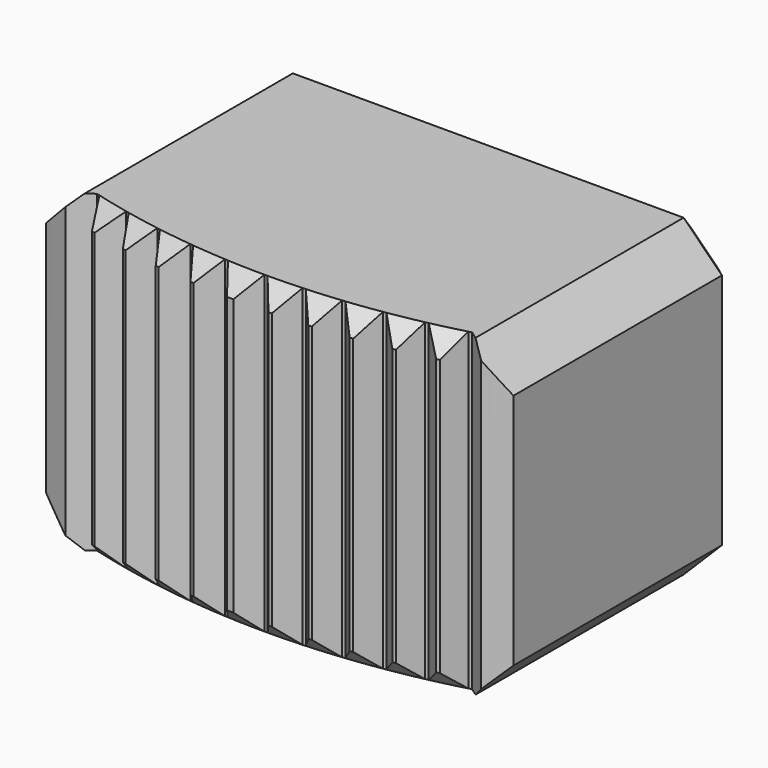
from build123d import *

# Parameters (mm, degrees)
F1_DEPTH = 4.1
F3_DEPTH = 0.75
F4_SIZE  = 1
F5_SIZE  = 0.5
F6_SIZE  = 0.5


# Not quite as in the source:
# - ends of sketch curves that miss each other by under 0.0002 mm in the source are joined


with BuildPart() as f1:
    # F0 (on Top) → F1 (new body, symmetric)
    with BuildSketch(Plane.XY):
        with BuildLine():
            Line((-6.1, 4.15), (-6.1, -3.15))
            ThreePointArc((-6.1, -3.15), (-5.7635565841, -3.2598963663), (-5.425135, -3.363541))
            Line((-5.425135, -3.363541), (-4.893695, -2.994868))
            Line((-4.893695, -2.994868), (-4.8153280581, -3.0160501894))
            Line((-4.8153280581, -3.0160501894), (-4.5419790581, -3.6022481894))
            ThreePointArc((-4.5419790581, -3.6022481894), (-4.5004913685, -3.6123533808), (-4.4589811968, -3.62236582))
            Line((-4.4589811968, -3.62236582), (-3.9475651968, -3.22638582))
            Line((-3.9475651968, -3.22638582), (-3.8681969582, -3.2434357798))
            Line((-3.8681969582, -3.2434357798), (-3.5645439582, -3.8145247798))
            ThreePointArc((-3.5645439582, -3.8145247798), (-3.5225838002, -3.822444913), (-3.4806060449, -3.8302712423))
            Line((-3.4806060449, -3.8302712423), (-2.9906150449, -3.4080672423))
            Line((-2.9906150449, -3.4080672423), (-2.9104630974, -3.4209427155))
            Line((-2.9104630974, -3.4209427155), (-2.5773370974, -3.9753557155))
            ThreePointArc((-2.5773370974, -3.9753557155), (-2.5350204133, -3.9810689039), (-2.4926910656, -3.9866874981))
            Line((-2.4926910656, -3.9866874981), (-2.0254680656, -3.5394184981))
            Line((-2.0254680656, -3.5394184981), (-1.9447520573, -3.5480806887))
            Line((-1.9447520573, -3.5480806887), (-1.5830670573, -4.0842996887))
            ThreePointArc((-1.5830670573, -4.0842996887), (-1.5405093729, -4.0877903631), (-1.4979439929, -4.0911859103))
            Line((-1.4979439929, -4.0911859103), (-1.0547689929, -3.6200769103))
            Line((-1.0547689929, -3.6200769103), (-0.9737100092, -3.624502302))
            Line((-0.9737100092, -3.624502302), (-0.5844580092, -4.141058302))
            ThreePointArc((-0.5844580092, -4.141058302), (-0.5001103826, -4.1434534303), (-0.415753, -4.1454759956))
            Line((-0.415753, -4.1454759956), (0, -3.6499999956))
            Line((0, -3.6499999956), (0.0811800024, -3.649823093))
            Line((0.0811800024, -3.649823093), (0.4990910024, -4.143480093))
            ThreePointArc((0.4990910024, -4.143480093), (0.541775859, -4.1423168954), (0.5844580091, -4.1410582978))
            Line((0.5844580091, -4.1410582978), (0.9737110091, -3.6245022978))
            Line((0.9737110091, -3.6245022978), (1.0547699921, -3.6200768997))
            Line((1.0547699921, -3.6200768997), (1.4979439921, -4.0911858997))
            ThreePointArc((1.4979439921, -4.0911858997), (1.5405098686, -4.087790312), (1.5830680495, -4.084299595))
            Line((1.5830680495, -4.084299595), (1.9447520495, -3.548080595))
            Line((1.9447520495, -3.548080595), (2.0254690462, -3.5394183512))
            Line((2.0254690462, -3.5394183512), (2.4926920462, -3.9866873512))
            ThreePointArc((2.4926920462, -3.9866873512), (2.5350213933, -3.9810687545), (2.5773380767, -3.9753555637))
            Line((2.5773380767, -3.9753555637), (2.9104640767, -3.4209425637))
            Line((2.9104640767, -3.4209425637), (2.9906160072, -3.4080670388))
            Line((2.9906160072, -3.4080670388), (3.4806070072, -3.8302710388))
            ThreePointArc((3.4806070072, -3.8302710388), (3.5225842788, -3.8224447977), (3.5645439535, -3.814524755))
            Line((3.5645439535, -3.814524755), (3.8681969535, -3.243435755))
            Line((3.8681969535, -3.243435755), (3.947566135, -3.2263855622))
            Line((3.947566135, -3.2263855622), (4.458982135, -3.6223655622))
            ThreePointArc((4.458982135, -3.6223655622), (4.5004922999, -3.6123531221), (4.5419799828, -3.6022479298))
            Line((4.5419799828, -3.6022479298), (4.8153289828, -3.0160499298))
            Line((4.8153289828, -3.0160499298), (4.893695989, -2.994867963))
            Line((4.893695989, -2.994867963), (5.425134989, -3.363540963))
            ThreePointArc((5.425134989, -3.363540963), (5.7635565104, -3.2598963467), (6.0999999321, -3.1500002293))
            Line((6.0999999321, -3.1500002293), (6.1, 4.15))
            Line((6.1, 4.15), (-6.1, 4.15))
        make_face()
    extrude(amount=F1_DEPTH, both=True)

    # F2 (on Top) → F3 (cut, symmetric)
    with BuildSketch(Plane.XY):
        with BuildLine():
            Line((2.9, 4.15), (-2.9, 4.15))
            Line((-2.9, 4.15), (-2.9, -0.85))
            ThreePointArc((-2.9, -0.85), (0, -1.85), (2.9, -0.85))
            Line((2.9, -0.85), (2.9, 4.15))
        make_face()
    extrude(amount=F3_DEPTH, both=True, mode=Mode.SUBTRACT)

    # F4
    f4_edges = [f1.edges().sort_by_distance(p)[0] for p in [
        (6.1, 0.5, -4.1),
        (-6.1, 0.5, -4.1),
        (-6.1, 0.5, 4.1),
        (6.1, 0.5, 4.1),
    ]]
    chamfer(f4_edges, length=F4_SIZE)

    # F5
    f5_edges = [f1.edges().sort_by_distance(p)[0] for p in [
        (0, 4.15, -4.1),
        (-5.6, 4.15, -3.6),
        (-6.1, 4.15, 0),
        (5.6, 4.15, -3.6),
        (6.1, 4.15, 0),
        (5.6, 4.15, 3.6),
        (0, 4.15, 4.1),
        (-5.6, 4.15, 3.6),
    ]]
    chamfer(f5_edges, length=F5_SIZE)

    # F6
    f6_edges = [f1.edges().sort_by_distance(p)[0] for p in [
        (-2.53502, -3.981069, -4.1),
        (-3.522584, -3.822445, -4.1),
        (-4.500491, -3.612353, -4.1),
        (-1.540509, -4.08779, -4.1),
        (-0.50011, -4.143453, -4.1),
        (0.541776, -4.142317, -4.1),
        (1.54051, -4.08779, -4.1),
        (2.535021, -3.981069, -4.1),
        (3.522584, -3.822445, -4.1),
        (4.500492, -3.612353, -4.1),
        (-4.500491, -3.612353, 4.1),
        (-3.522584, -3.822445, 4.1),
        (-2.53502, -3.981069, 4.1),
        (-1.540509, -4.08779, 4.1),
        (-0.50011, -4.143453, 4.1),
        (0.541776, -4.142317, 4.1),
        (1.54051, -4.08779, 4.1),
        (2.535021, -3.981069, 4.1),
        (3.522584, -3.822445, 4.1),
        (4.500492, -3.612353, 4.1),
    ]]
    chamfer(f6_edges, length=F6_SIZE)


solid = f1.part
